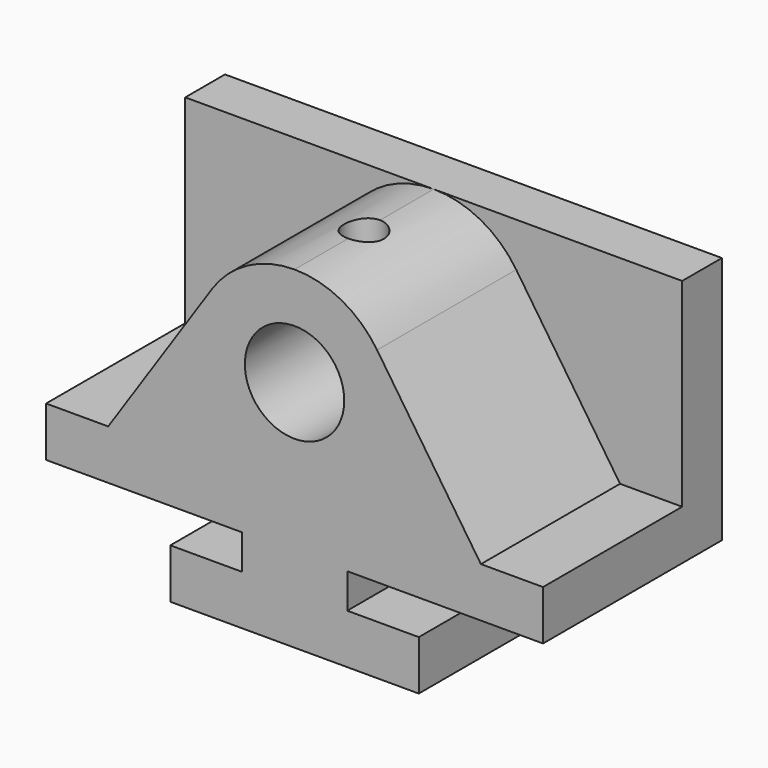
from build123d import *

# Parameters (mm, degrees)
F1_DEPTH = 57.15
F2_R     = 12.7
F3_DEPTH = 44.45
F4_R     = 5.08
F5_DEPTH = 13.7758108493


# Not quite as in the source:
# - ends of sketch curves that miss each other by under 0.0002 mm in the source are joined


with BuildPart() as f1:
    # F0 (on Front) → F1 (new body)
    with BuildSketch(Plane.XZ):
        Polygon((-31.75, 0), (31.75, 0), (31.75, 12.7), (13.4683688998, 12.7), (13.4683688998, 21.59), (63.5, 21.59), (63.5, 85.09), (-63.5, 85.09), (-63.5, 21.59), (-13.4683688998, 21.59), (-13.4683688998, 12.7), (-31.75, 12.7), align=None)
    extrude(amount=-F1_DEPTH)

    # F2 (on face) → F3 (cut)
    with BuildSketch(Plane.XZ):
        with BuildLine():
            Line((0, 85.09), (-63.5, 85.09))
            Line((-63.5, 85.09), (-63.5, 34.29))
            Line((-63.5, 34.29), (-47.625, 34.29))
            Line((-47.625, 34.29), (-21.0934436414, 73.8401851094))
            ThreePointArc((-21.0934436414, 73.8401851094), (-11.9529513968, 82.101783869), (0, 85.09))
        make_face()
        with Locations((0, 59.69)):
            Circle(F2_R)
        with BuildLine():
            Line((63.5, 85.09), (0, 85.09))
            ThreePointArc((0, 85.09), (11.9529513968, 82.101783869), (21.0934436414, 73.8401851094))
            Line((21.0934436414, 73.8401851094), (47.625, 34.29))
            Line((47.625, 34.29), (63.5, 34.29))
            Line((63.5, 34.29), (63.5, 85.09))
        make_face()
    extrude(amount=-F3_DEPTH, mode=Mode.SUBTRACT)

    # F4 (on face) → F5 (cut, through all)
    with BuildSketch(Plane.XY.offset(85.09)):
        with Locations((-0.0332157188, 22.225)):
            Circle(F4_R)
    extrude(amount=-F5_DEPTH, mode=Mode.SUBTRACT)


solid = f1.part
